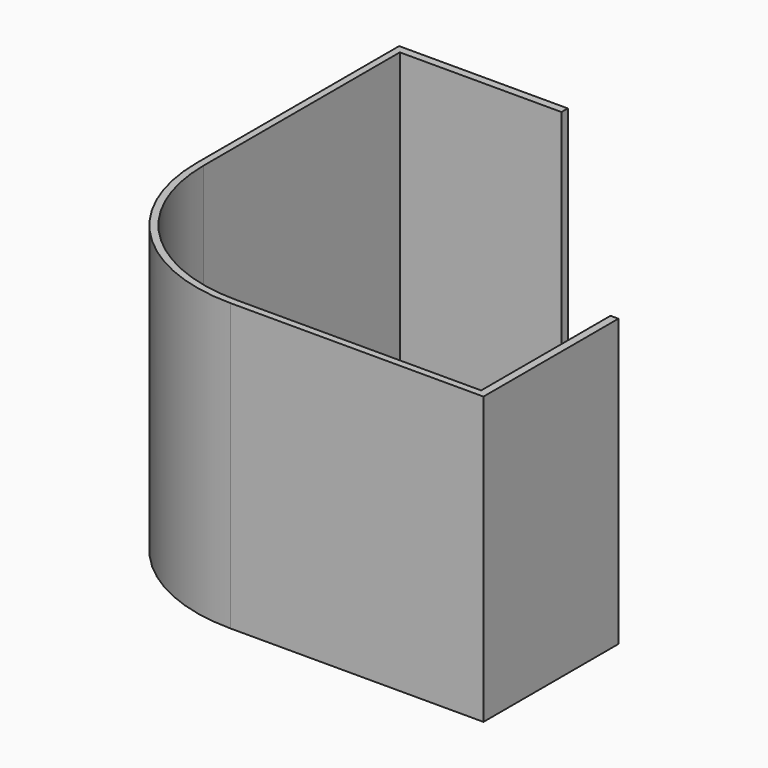
from build123d import *

# Parameters (mm, degrees)
F0_W     = 584.2
F0_H     = 28.575
F0_W_2   = 28.575
F0_H_2   = 584.2
F1_DEPTH = 1035.05


with BuildPart() as f1:
    # F0 (on Top) → F1 (new body)
    with BuildSketch(Plane.XY):
        with Locations((12.7, 747.7125)):
            Rectangle(F0_W, F0_H)
        Polygon((-279.4, 733.425), (-279.4, 762), (-304.8, 762), (-304.8, -152.4), (-279.4, -152.4), align=None)
        with BuildLine():
            Line((-279.4, -152.4), (-304.8, -152.4))
            ThreePointArc((-304.8, -152.4), (-126.2522938113, -583.4522938113), (304.8, -762))
            Line((304.8, -762), (304.8, -736.6))
            ThreePointArc((304.8, -736.6), (-108.2917815692, -565.4917815692), (-279.4, -152.4))
        make_face()
        Polygon((304.8, -736.6), (304.8, -762), (1219.2, -762), (1219.2, -736.6), (1190.625, -736.6), align=None)
        with Locations((1204.9125, -444.5)):
            Rectangle(F0_W_2, F0_H_2)
    extrude(amount=F1_DEPTH)


solid = f1.part
